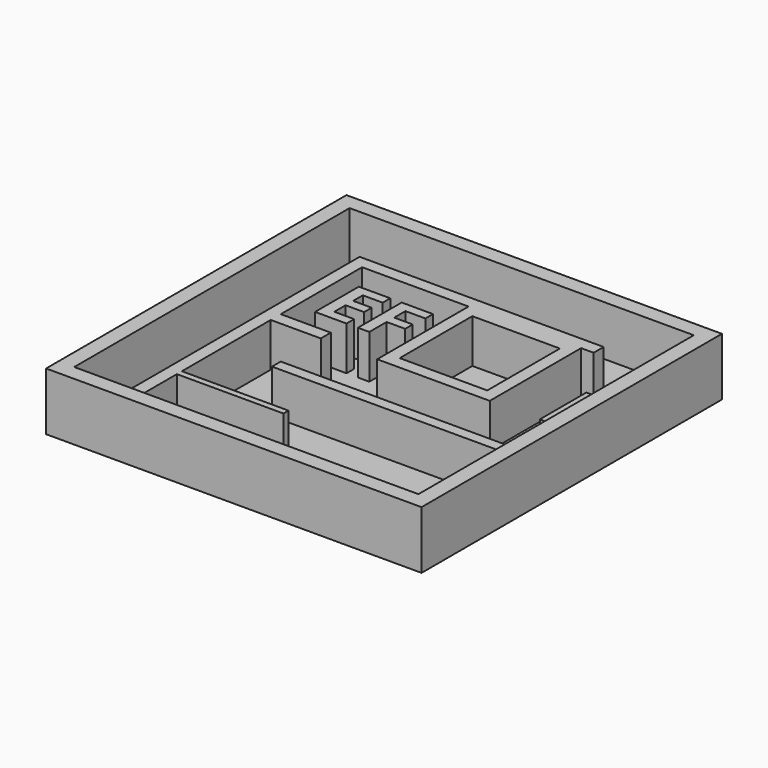
from build123d import *

# Parameters (mm, degrees)
F0_W         = 38.1
F0_H         = 38.1
F1_DEPTH     = 0.79375
F2_W         = 38.1
F2_H         = 38.1
F2_W_2       = 34.925
F2_H_2       = 34.925
F3_DEPTH     = 5.08
F4_R         = 1.27
F5_DEPTH     = 0.396875
F4_W         = 8.8854621942
F4_H         = 9.2124652583
F4_W_2       = 23.495
F4_H_2       = 1.1114065551
F4_W_3       = 5.08
F4_H_3       = 1.27
F4_W_4       = 10.8201340951
F4_H_4       = 0.6364464461
F4_W_5       = 1.27
F4_H_5       = 5.8953870241
F6_DEPTH     = 4.445
F4_TEXT_SIZE = 7.7696281045
F7_DEPTH     = 4.445


# Not quite as in the source:
# - Text() gives the source's letters only with a copy of the font that has no kerning and outlines rounded to 1/6400 em; it was checked with that copy


with BuildPart() as f1:
    # F0 (on Top) → F1 (new body)
    with BuildSketch(Plane.XY):
        with Locations((3.31386365, -3.3247117253)):
            Rectangle(F0_W, F0_H)
    extrude(amount=F1_DEPTH)

    # F2 (on face) → F3 (join)
    with BuildSketch(Plane.XY.offset(0.79375)):
        with Locations((3.31386365, -3.3247117253)):
            Rectangle(F2_W, F2_H)
        with Locations((3.31386365, -3.3247117253)):
            Rectangle(F2_W_2, F2_H_2, mode=Mode.SUBTRACT)
    extrude(amount=F3_DEPTH)

    # F4 (on face) → F5 (cut)
    with BuildSketch(Plane.XY.offset(0.79375)):
        with Locations((-11.60863635, -15.5707597733)):
            Circle(F4_R)
        with Locations((-4.1899718344, -18.2472117253)):
            Circle(F4_R)
    extrude(amount=-F5_DEPTH, mode=Mode.SUBTRACT)

    # F4 (on face) → F6 (join)
    with BuildSketch(Plane.XY.offset(0.79375)):
        Polygon((-9.06863635, 9.0577882747), (-9.06863635, -20.7872117253), (-7.79863635, -20.7872117253), (-7.79863635, -15.7072117253), (-7.79863635, -15.0707652792), (-7.79863635, -3.7993587241), (-7.79863635, -2.5293587241), (-7.79863635, 7.7877882747), (3.0009014557, 7.7877882747), (3.0009014557, -3.7993587241), (14.42636365, -3.7993587241), (14.42636365, 7.7877882747), (15.69636365, 7.7877882747), (15.69636365, 9.0577882747), (-7.79863635, 9.0577882747), align=None)
        with Locations((8.7136325528, 2.076873905)):
            Rectangle(F4_W, F4_H, mode=Mode.SUBTRACT)
        with Locations((9.02886365, -9.4350620017)):
            Rectangle(F4_W_2, F4_H_2)
        with Locations((-5.25863635, -3.1643587241)):
            Rectangle(F4_W_3, F4_H_3)
        with Locations((-2.3885693025, -15.3889885023)):
            Rectangle(F4_W_4, F4_H_4)
        with Locations((20.14136365, -0.8516652121)):
            Rectangle(F4_W_5, F4_H_5)
    extrude(amount=F6_DEPTH)

    # F4 (on face) → F7 (join)
    with BuildSketch(Plane.XY.offset(0.79375)):
        with Locations((-6.6172149964, -0.5289169494)):
            Text('EF', F4_TEXT_SIZE, font='Open Sans', font_style=FontStyle.BOLD, text_align=(TextAlign.LEFT, TextAlign.BOTTOM))
    extrude(amount=F7_DEPTH)


solid = f1.part
